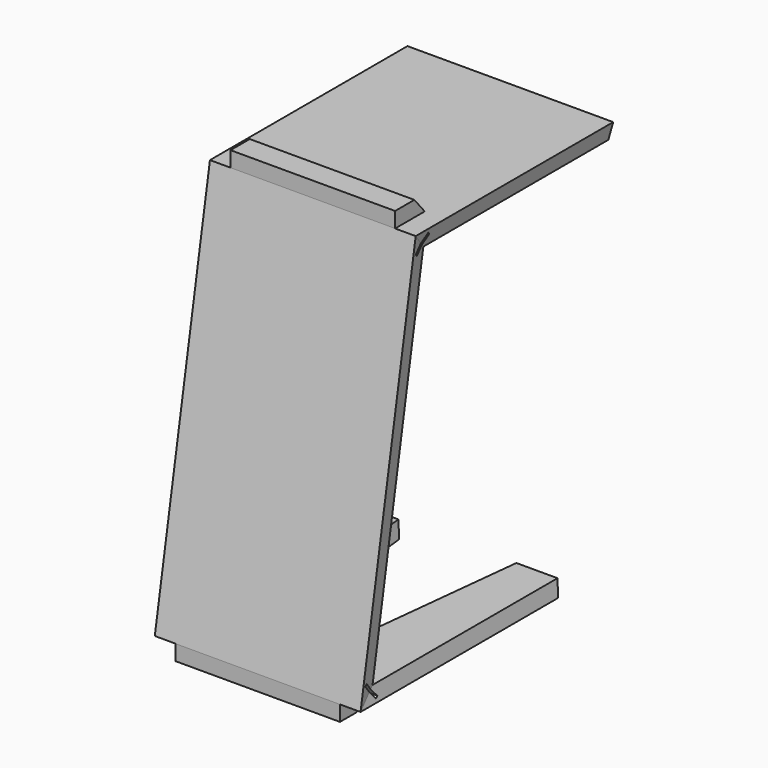
from build123d import *

# Parameters (mm, degrees)
F1_DEPTH      = 127
F2_SIZE2      = 3.359019
F2_SIZE       = 19.04999
F3_SIZE2      = 3.359019
F3_SIZE       = 19.04999
F5_DEPTH      = 19.051
F5_TAPER      = 10
F7_DEPTH      = 127.0010001
F7_DEPTH_BACK = 127.0010001
F9_DEPTH      = 101.6


# Not quite as in the source:
# - a fillet or chamfer is up to 0.001 mm smaller than in the source, because OpenCascade refuses the exact size


with BuildPart() as f1:
    # F0 (on Right) → F1 (new body, symmetric)
    with BuildSketch(Plane.YZ):
        Polygon((22.7029059389, 19.05), (0, 0), (304.8, 0), (308.1590289825, 19.05), align=None)
        Polygon((85.0954008899, 482.6), (0, 0), (22.7029059389, 19.05), (101.0802488638, 463.55), align=None)
        Polygon((389.8954008899, 482.6), (85.0954008899, 482.6), (101.0802488638, 463.55), (386.5363719074, 463.55), align=None)
    extrude(amount=F1_DEPTH, both=True)

    # F2 (size 19.05 and 3.3590289825 in the source; OpenCascade refuses exactly that, so slightly less here)
    f2_edges = [f1.edges().sort_by_distance(p)[0] for p in [
        (127, 243.80831, 463.55),
        (127, 61.891577, 241.3),
        (127, 165.430967, 19.05),
    ]]
    f2_side = f1.faces().sort_by_distance((127, 152.4, 6.204202))[0]
    chamfer(f2_edges, length=F2_SIZE, length2=F2_SIZE2, reference=f2_side)

    # F3 (size 19.05 and 3.3590289825 in the source; OpenCascade refuses exactly that, so slightly less here)
    f3_edges = [f1.edges().sort_by_distance(p)[0] for p in [
        (-127, 243.80831, 463.55),
        (-127, 61.891577, 241.3),
        (-127, 165.430967, 19.05),
    ]]
    f3_side = f1.faces().sort_by_distance((-127, 152.4, 6.204202))[0]
    chamfer(f3_edges, length=F3_SIZE, length2=F3_SIZE2, reference=f3_side)

    # F4 (on face) → F5 (cut, through all)
    with BuildSketch(Plane.XY.offset(19.05)):
        Polygon((47.4409710175, 73.5029059389), (72.8409710175, 308.1590289825), (0, 308.1590289825), (-72.8409710175, 308.1590289825), (-47.4409710175, 73.5029059389), (0, 73.5029059389), align=None)
    extrude(amount=-F5_DEPTH, taper=F5_TAPER, mode=Mode.SUBTRACT)

    # F6 (on Right) → F7 (cut, two sides)
    with BuildSketch(Plane.YZ) as f7_sk:
        Polygon((86.2493577843, 461.4670751242), (88.2902084451, 459.0348840173), (107.7477373003, 475.3616893034), (105.7068866396, 477.7938804103), align=None)
        Polygon((27.2180219216, 6.2599595813), (10.8912166355, 25.7174884365), (8.4590255286, 23.6766377757), (24.7858308147, 4.2191089205), align=None)
    extrude(amount=-F7_DEPTH, mode=Mode.SUBTRACT)
    extrude(f7_sk.sketch, amount=F7_DEPTH_BACK, mode=Mode.SUBTRACT)


with BuildPart() as f9:
    # F8 (on Right) → F9 (new body, symmetric)
    with BuildSketch(Plane.YZ):
        Polygon((114.7936259095, 501.65), (85.0954008899, 501.65), (85.0954008899, 482.6), (130.7784738835, 482.6), align=None)
    extrude(amount=F9_DEPTH, both=True)


with BuildPart() as f9b:
    # F8 (on Right) → F9, piece 2 (new body, symmetric)
    with BuildSketch(Plane.YZ):
        Polygon((47.6699605102, 0), (0, 0), (0, -19.05), (24.9670545713, -19.05), align=None)
    extrude(amount=F9_DEPTH, both=True)


solid = Compound([f1.part, f9.part, f9b.part])
